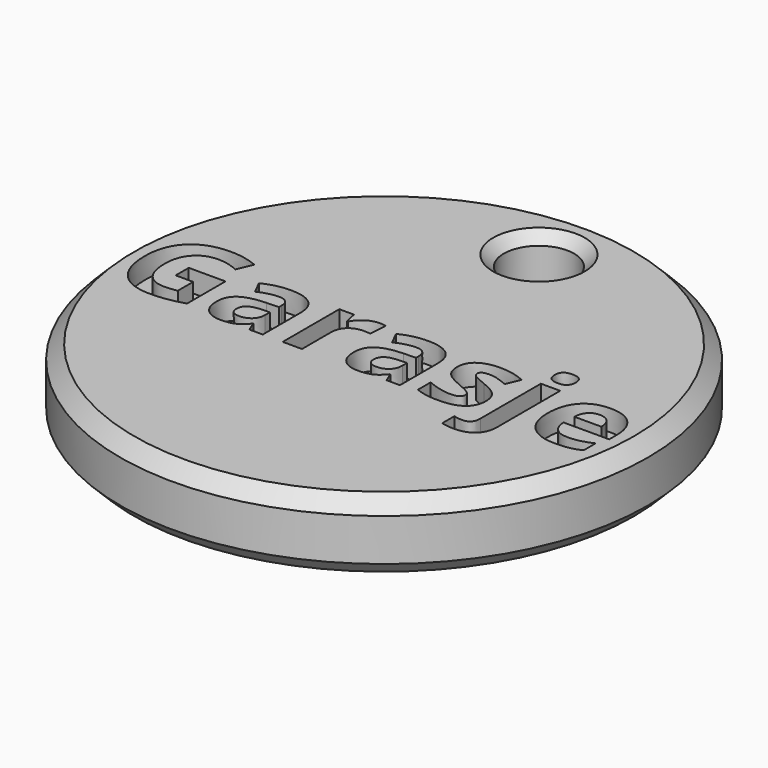
from build123d import *

# Parameters (mm, degrees)
F0_R         = 15
F0_R_2       = 2
F1_DEPTH     = 4
F2_TEXT_SIZE = 7.366300818
F3_DEPTH     = 1.2
F4_SIZE      = 0.8
F5_SIZE      = 0.6


# Not quite as in the source:
# - Text() gives the source's letters only with a copy of the font that has no kerning and outlines rounded to 1/6400 em; it was checked with that copy


with BuildPart() as f1:
    # F0 (on Top) → F1 (new body)
    with BuildSketch(Plane.XY):
        Circle(F0_R)
        with Locations((0, 11)):
            Circle(F0_R_2, mode=Mode.SUBTRACT)
    extrude(amount=F1_DEPTH)

    # F2 (on face) → F3 (cut)
    with BuildSketch(Plane.XY.offset(4)):
        with Locations((-14, -2.6518682945)):
            Text('Garasje', F2_TEXT_SIZE, font='Open Sans', font_style=FontStyle.BOLD, text_align=(TextAlign.LEFT, TextAlign.BOTTOM))
    extrude(amount=-F3_DEPTH, mode=Mode.SUBTRACT)

    # F4
    f4_edges = [f1.edges().sort_by_distance(p)[0] for p in [
        (-15, 0, 4),
        (-15, 0, 0),
    ]]
    chamfer(f4_edges, length=F4_SIZE)

    # F5
    f5_edges = [f1.edges().sort_by_distance(p)[0] for p in [
        (-2, 11, 4),
        (-2, 11, 0),
    ]]
    chamfer(f5_edges, length=F5_SIZE)


solid = f1.part
